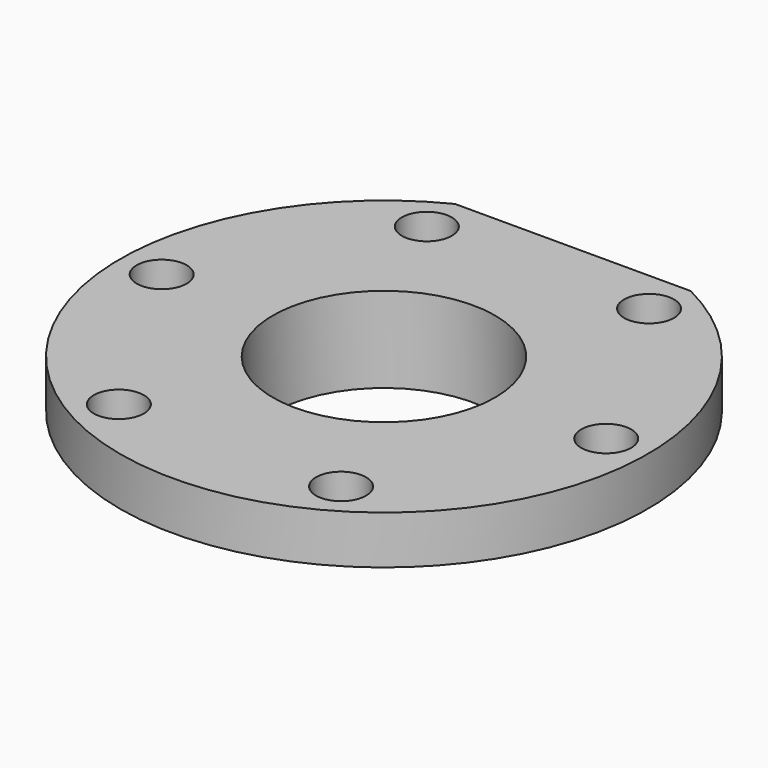
from build123d import *

# Parameters (mm, degrees)
F0_R            = 47.5
F1_DEPTH        = 8.7
F2_R            = 34
F3_DEPTH        = 15.4
F5_DEPTH        = 15.401
F6_R            = 20
F7_DEPTH        = 15.401
F9_D            = 9
F9_COPIES_COUNT = 6


# Not quite as in the source:
# - a pattern or mirror of a feature is missing from the dataset's text; its kind, count and spacing are read off the source's solid


with BuildPart() as f1:
    # F0 (on Top) → F1 (new body)
    with BuildSketch(Plane.XY):
        Circle(F0_R)
    extrude(amount=-F1_DEPTH)

    # F2 (on face) → F3 (join)
    with BuildSketch(Plane.XY):
        Circle(F2_R)
    extrude(amount=-F3_DEPTH)

    # F4 (on face) → F5 (cut, through all)
    with BuildSketch(Plane.XY):
        with BuildLine():
            Line((-21.2132034356, 42.5), (21.2132034356, 42.5))
            ThreePointArc((21.2132034356, 42.5), (0, 47.5), (-21.2132034356, 42.5))
        make_face()
    extrude(amount=-F5_DEPTH, mode=Mode.SUBTRACT)

    # F6 (on face) → F7 (cut, through all)
    with BuildSketch(Plane.XY):
        Circle(F6_R)
    extrude(amount=-F7_DEPTH, mode=Mode.SUBTRACT)

    # F9 (through all)
    with Locations(Plane.XY):
        with Locations((-40, 0)):
            f9 = Hole(F9_D / 2)

    # F9_copies: F9 ×6 about axis
    f9_copies_axis = Axis((0, 0, 0), (0, 0, 1))
    for i in range(1, F9_COPIES_COUNT):
        add(f9.rotate(f9_copies_axis, i * 360 / F9_COPIES_COUNT), mode=Mode.SUBTRACT)


solid = f1.part
